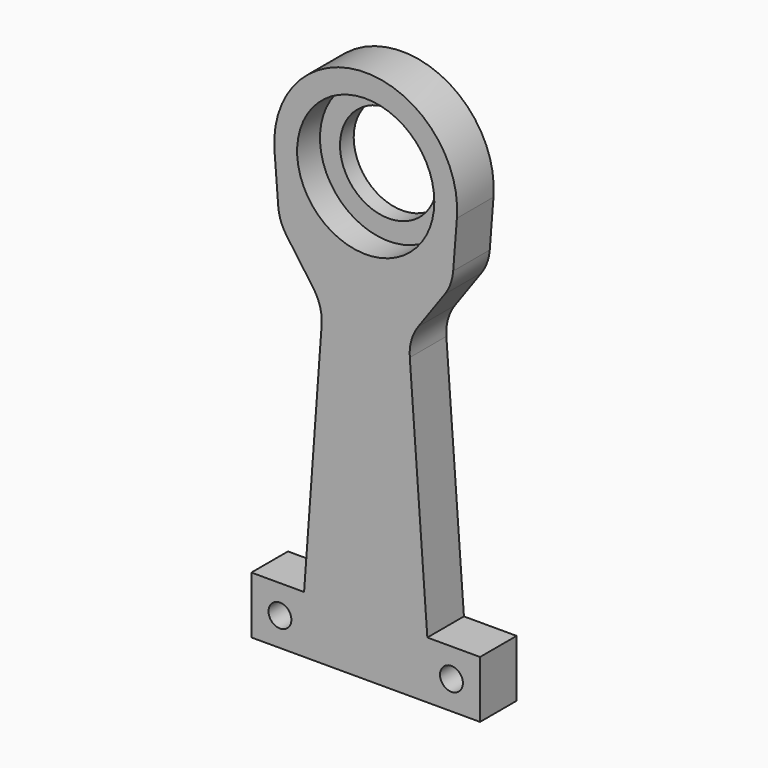
from build123d import *

# Parameters (mm, degrees)
F0_R     = 12
F1_DEPTH = 8
F3_DEPTH = 25
F4_R     = 8
F5_R     = 12
F5_R_2   = 8.5
F6_DEPTH = 3
F7_R     = 2
F8_DEPTH = 25


with BuildPart() as f1:
    # F0 (on Front) → F1 (new body)
    with BuildSketch(Plane.XZ):
        with BuildLine():
            Line((10.7804718609, -67.5), (15.9514905981, -1.2449689551))
            ThreePointArc((15.9514905981, -1.2449689551), (0, 16), (-15.9514905981, -1.2449689551))
            Line((-15.9514905981, -1.2449689551), (-10.7804718609, -67.5))
            Line((-10.7804718609, -67.5), (-20, -67.5))
            Line((-20, -67.5), (-20, -77.5))
            Line((-20, -77.5), (-10, -77.5))
            Line((-10, -77.5), (10, -77.5))
            Line((10, -77.5), (20, -77.5))
            Line((20, -77.5), (20, -67.5))
            Line((20, -67.5), (10.7804718609, -67.5))
        make_face()
        Circle(F0_R, mode=Mode.SUBTRACT)
    extrude(amount=F1_DEPTH)

    # F2 (on face) → F3 (cut)
    with BuildSketch(Plane(origin=(0, 0, 0), x_dir=(-1, 0, 0), z_dir=(0, 1, 0))):
        Polygon((-7.5, -22.5), (-15.1268365117, -11.8110652832), (-10.7804718609, -67.5), align=None)
        Polygon((10.7804718609, -67.5), (15.1268365117, -11.8110652832), (7.5, -22.5), align=None)
    extrude(amount=-F3_DEPTH, mode=Mode.SUBTRACT)

    # F4
    f4_edges = [f1.edges().sort_by_distance(p)[0] for p in [
        (-7.5, -4, -22.5),
        (-15.126837, -4, -11.811065),
        (15.126837, -4, -11.811065),
        (7.5, -4, -22.5),
    ]]
    fillet(f4_edges, radius=F4_R)

    # F5 (on face) → F6 (join)
    with BuildSketch(Plane(origin=(0, 0, 0), x_dir=(-1, 0, 0), z_dir=(0, 1, 0))):
        with BuildLine():
            Line((20, -67.5), (10.7804718609, -67.5))
            Line((10.7804718609, -67.5), (7.7098565421, -25.3787152568))
            ThreePointArc((7.7098565421, -25.3787152568), (7.9860060263, -22.6363328806), (9.1764777393, -20.150433298))
            Line((9.1764777393, -20.150433298), (13.8361972063, -13.6198832981))
            ThreePointArc((13.8361972063, -13.6198832981), (14.8422105338, -11.7075498191), (15.2997366254, -9.5957373215))
            Line((15.2997366254, -9.5957373215), (15.9514905981, -1.2449689551))
            ThreePointArc((15.9514905981, -1.2449689551), (0, 16), (-15.9514905981, -1.2449689551))
            Line((-15.9514905981, -1.2449689551), (-15.2997366254, -9.5957373215))
            ThreePointArc((-15.2997366254, -9.5957373215), (-14.8422105338, -11.7075498191), (-13.8361972063, -13.6198832981))
            Line((-13.8361972063, -13.6198832981), (-9.1764777393, -20.150433298))
            ThreePointArc((-9.1764777393, -20.150433298), (-7.9860060263, -22.6363328806), (-7.7098565421, -25.3787152568))
            Line((-7.7098565421, -25.3787152568), (-10.7804718609, -67.5))
            Line((-10.7804718609, -67.5), (-20, -67.5))
            Line((-20, -67.5), (-20, -77.5))
            Line((-20, -77.5), (20, -77.5))
            Line((20, -77.5), (20, -67.5))
        make_face()
        Circle(F5_R, mode=Mode.SUBTRACT)
        Circle(F5_R)
        Circle(F5_R_2, mode=Mode.SUBTRACT)
    extrude(amount=-F6_DEPTH)

    # F7 (on face) → F8 (cut)
    with BuildSketch(Plane.XZ.offset(8)):
        with Locations((-15, -72.5)):
            Circle(F7_R)
        with Locations((15, -72.5)):
            Circle(F7_R)
    extrude(amount=-F8_DEPTH, mode=Mode.SUBTRACT)


solid = f1.part
